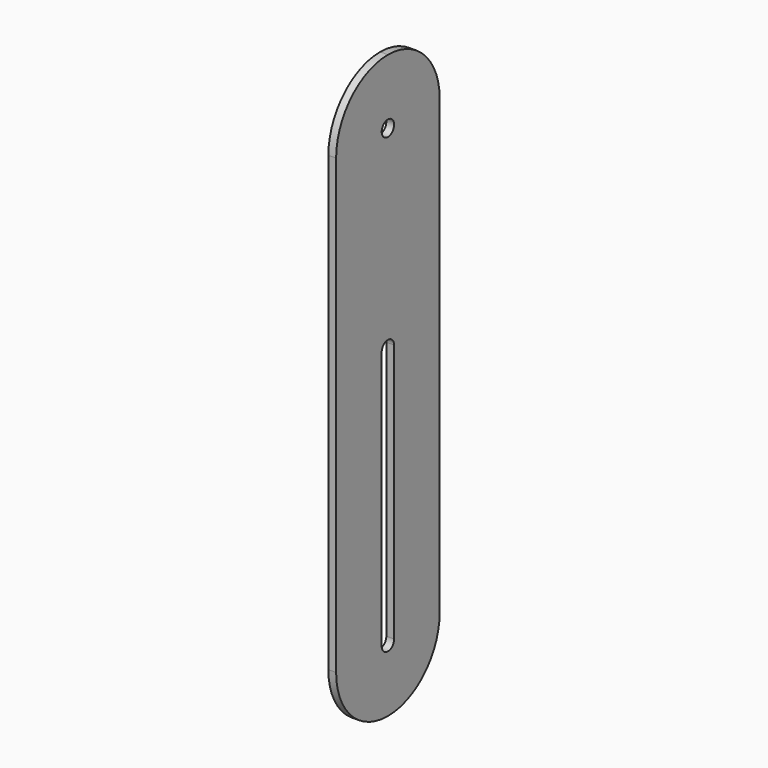
from build123d import *

# Parameters (mm, degrees)
F0_W        = 50
F0_H        = 400
F1_DEPTH    = 3
F2_T1_DEPTH = 128
F3_R        = 3
F4_DEPTH    = 25
F6_DEPTH    = 25
F8_DEPTH    = 25


# Not quite as in the source:
# - a fillet or chamfer that OpenCascade refuses, or shapes differently, is made with other operations: its cross-section is extruded or revolved along the edge and cut away or added


with BuildPart() as f1:
    # F0 (on Right) → F1 (new body)
    with BuildSketch(Plane.YZ):
        Rectangle(F0_W, F0_H)
    extrude(amount=F1_DEPTH)

    # F2: fillet of radius 25 on 4 edges, made by hand

    # F2_s2 → F2_t1 (cut)
    with BuildSketch(Plane.YZ.offset(-62.5)):
        with BuildLine():
            ThreePointArc((0, 200), (-17.6776695297, 192.6776695297), (-25, 175))
            Line((-25, 175), (-25, 200))
            Line((-25, 200), (0, 200))
        make_face()
        with BuildLine():
            ThreePointArc((-25, -175), (-17.6776695297, -192.6776695297), (0, -200))
            Line((0, -200), (-25, -200))
            Line((-25, -200), (-25, -175))
        make_face()
        with BuildLine():
            ThreePointArc((25, 175), (17.6776695297, 192.6776695297), (0, 200))
            Line((0, 200), (25, 200))
            Line((25, 200), (25, 175))
        make_face()
        with BuildLine():
            ThreePointArc((25, -175), (17.6776695297, -192.6776695297), (0, -200))
            Line((0, -200), (25, -200))
            Line((25, -200), (25, -175))
        make_face()
    extrude(amount=F2_T1_DEPTH, mode=Mode.SUBTRACT)

    # F3 (on face) → F4 (cut)
    with BuildSketch(Plane.YZ.offset(3)):
        with Locations((0, 175)):
            Circle(F3_R)
    extrude(amount=-F4_DEPTH, mode=Mode.SUBTRACT)

    # F5 (on face) → F6 (cut)
    with BuildSketch(Plane.YZ.offset(3)):
        with BuildLine():
            ThreePointArc((-3, 100), (0, 97), (3, 100))
            ThreePointArc((3, 100), (0, 103), (-3, 100))
        make_face()
        with BuildLine():
            Line((3, 0), (3, 100))
            ThreePointArc((3, 100), (0, 97), (-3, 100))
            Line((-3, 100), (-3, 0))
            ThreePointArc((-3, 0), (0, 3), (3, 0))
        make_face()
        with BuildLine():
            ThreePointArc((-3, 0), (0, -3), (3, 0))
            ThreePointArc((3, 0), (0, 3), (-3, 0))
        make_face()
    extrude(amount=-F6_DEPTH, mode=Mode.SUBTRACT)

    # F7 (on face) → F8 (cut)
    with BuildSketch(Plane.YZ.offset(3)):
        with BuildLine():
            ThreePointArc((25, 0), (0, -25), (-25, 0))
            Line((-25, 0), (-25, -175))
            ThreePointArc((-25, -175), (0, -200), (25, -175))
            Line((25, -175), (25, 0))
        make_face()
    extrude(amount=-F8_DEPTH, mode=Mode.SUBTRACT)


solid = f1.part
